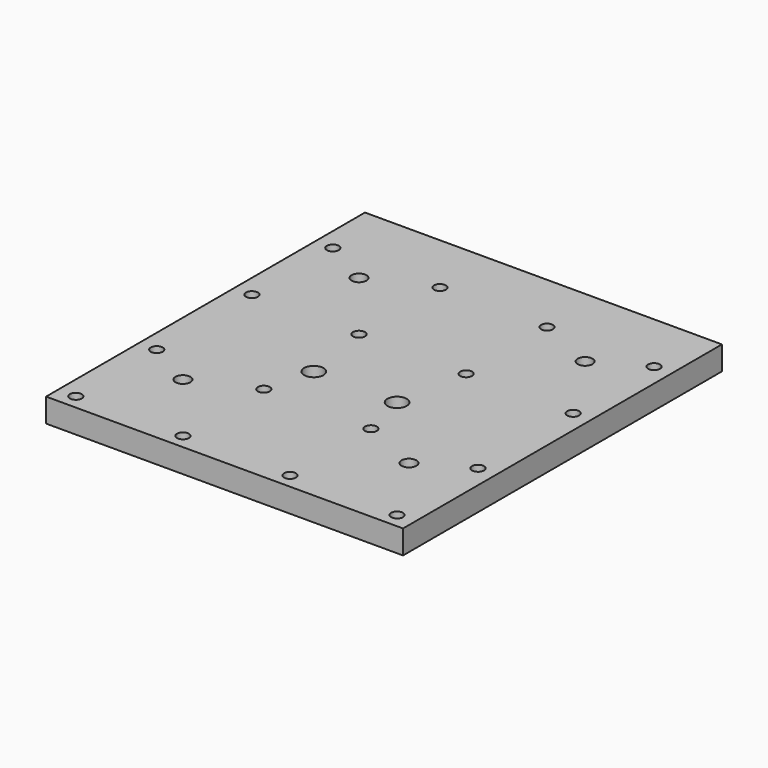
from build123d import *

# Parameters (mm, degrees)
F0_W             = 120
F0_H             = 150
F1_DEPTH         = 8
F2_R             = 2
F3_DEPTH         = 8
F3_COPIES_COUNT  = 3
F3_COPIES_PITCH  = 36
F3_COPIES2_COUNT = 2
F3_COPIES2_PITCH = 103.247276
F4_R             = 3.25
F4_W             = 120
F4_H             = 16
F4_R_2           = 2.5
F5_DEPTH         = 8


# Not quite as in the source:
# - a pattern or mirror of a feature is missing from the dataset's text; its kind, count and spacing are read off the source's solid


with BuildPart() as f1:
    # F0 (on Top) → F1 (new body)
    with BuildSketch(Plane.XY):
        Rectangle(F0_W, F0_H)
    extrude(amount=F1_DEPTH)

    # F2 (on face) → F3 (cut, through all)
    with BuildSketch(Plane.XY.offset(8)):
        with Locations((-54, 54)):
            Circle(F2_R)
        with Locations((-18, 54)):
            Circle(F2_R)
        with Locations((-18, 20)):
            Circle(F2_R)
        with Locations((-54, 20)):
            Circle(F2_R)
    f3 = extrude(amount=-F3_DEPTH, mode=Mode.SUBTRACT)

    # F3_copies: F3 ×3
    with Locations(*[(i * F3_COPIES_PITCH, 0, 0) for i in range(1, F3_COPIES_COUNT)]):
        add(f3, mode=Mode.SUBTRACT)

    # F3_copies1: F3 across plane
    add(f3.mirror(Plane(origin=(0, 0, 0), x_dir=(0, 0, -1), z_dir=(0, -1, 0))), mode=Mode.SUBTRACT)

    # F3_copies2: F3 ×2
    with Locations(*[Vector(0.6973549598, -0.7167259309, 0) * (i * F3_COPIES2_PITCH) for i in range(1, F3_COPIES2_COUNT)]):
        add(f3, mode=Mode.SUBTRACT)

    # F4 (on face) → F5 (cut, through all)
    with BuildSketch(Plane.XY.offset(8)):
        with Locations((-14, -4)):
            Circle(F4_R)
        with Locations((14, -4)):
            Circle(F4_R)
        with Locations((0, -67)):
            Rectangle(F4_W, F4_H)
        with Locations((38, -29)):
            Circle(F4_R_2)
        with Locations((38, 45)):
            Circle(F4_R_2)
        with Locations((-38, 45)):
            Circle(F4_R_2)
        with Locations((-38, -29)):
            Circle(F4_R_2)
    extrude(amount=-F5_DEPTH, mode=Mode.SUBTRACT)


solid = f1.part
